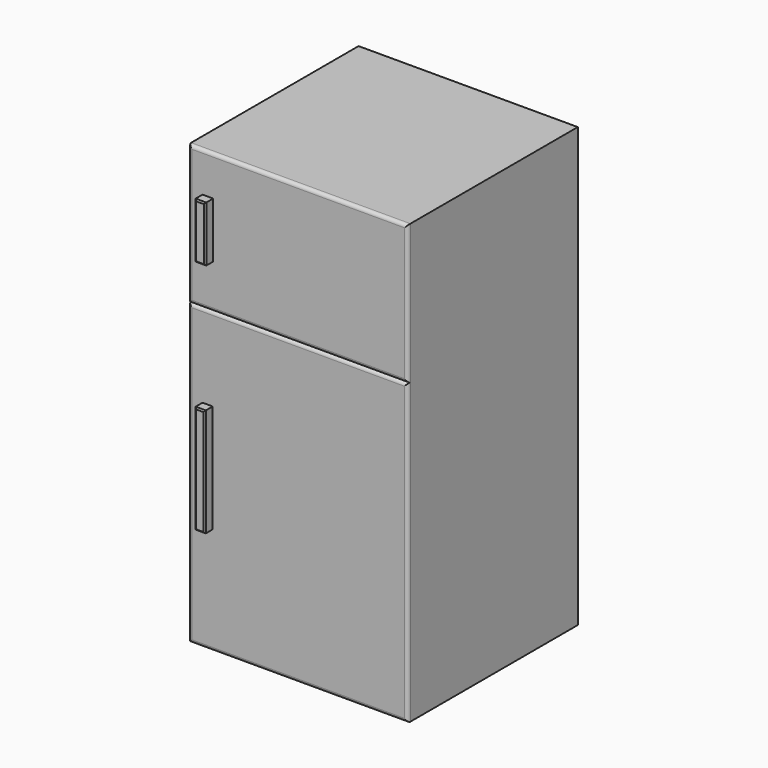
from build123d import *

# Parameters (mm, degrees)
F0_W      = 838.2
F0_H      = 762
F1_DEPTH  = 1676.4
F2_W      = 838.2
F2_H      = 533.4
F2_W_2    = 38.1
F2_H_2    = 203.2
F3_DEPTH  = 50.8
F4_R      = 12.7
F5_DEPTH  = 50.8
F6_R      = 12.69999
F7_W      = 40.6822860241
F7_H      = 212.2554779053
F8_DEPTH  = 38.1
F9_SIZE   = 5.08
F10_W     = 38.9135181904
F10_H     = 413.8980805874
F11_DEPTH = 38.1
F12_SIZE  = 5.08


# Not quite as in the source:
# - a fillet or chamfer is up to 0.001 mm smaller than in the source, because OpenCascade refuses the exact size


with BuildPart() as f1:
    # F0 (on Top) → F1 (new body)
    with BuildSketch(Plane.XY):
        Rectangle(F0_W, F0_H)
    extrude(amount=F1_DEPTH)

    # F2 (on face) → F3 (join)
    with BuildSketch(Plane.XZ.offset(381)):
        with Locations((0, 1409.7)):
            Rectangle(F2_W, F2_H)
        with Locations((-346.277383852, 1415.0833574295)):
            Rectangle(F2_W_2, F2_H_2, mode=Mode.SUBTRACT)
        with Locations((-346.277383852, 1415.0833574295)):
            Rectangle(F2_W_2, F2_H_2)
    extrude(amount=F3_DEPTH)

    # F4
    f4_edges = [f1.edges().sort_by_distance(p)[0] for p in [
        (0, -431.8, 1676.4),
        (-419.1, -431.8, 1409.7),
        (0, -431.8, 1143),
        (419.1, -431.8, 1409.7),
    ]]
    fillet(f4_edges, radius=F4_R)

    # F5 (add): a face of the model
    f5_faces = [f1.faces().sort_by_distance(p)[0] for p in [
        (0, -381, 571.5),
    ]]
    extrude(f5_faces, amount=F5_DEPTH)

    # F6 (radius 12.7 in the source; OpenCascade refuses exactly that, so slightly less here)
    f6_edges = [f1.edges().sort_by_distance(p)[0] for p in [
        (0, -431.8, 0),
        (419.1, -431.8, 571.5),
        (0, -431.8, 1143),
        (-419.1, -431.8, 571.5),
    ]]
    fillet(f6_edges, radius=F6_R)

    # F7 (on face) → F8 (join)
    with BuildSketch(Plane.XZ.offset(431.8)):
        with Locations((-345.143482089, 1418.1935787201)):
            Rectangle(F7_W, F7_H)
    extrude(amount=F8_DEPTH)

    # F9
    f9_edges = [f1.edges().sort_by_distance(p)[0] for p in [
        (-345.143482, -469.9, 1524.321318),
        (-365.484625, -469.9, 1418.193579),
        (-345.143482, -469.9, 1312.06584),
        (-324.802339, -469.9, 1418.193579),
    ]]
    chamfer(f9_edges, length=F9_SIZE)

    # F10 (on face) → F11 (join)
    with BuildSketch(Plane.XZ.offset(431.8)):
        with Locations((-346.0278660059, 616.92930758)):
            Rectangle(F10_W, F10_H)
    extrude(amount=F11_DEPTH)

    # F12
    f12_edges = [f1.edges().sort_by_distance(p)[0] for p in [
        (-346.027866, -469.9, 823.878348),
        (-365.484625, -469.9, 616.929308),
        (-346.027866, -469.9, 409.980267),
        (-326.571107, -469.9, 616.929308),
    ]]
    chamfer(f12_edges, length=F12_SIZE)


solid = f1.part
